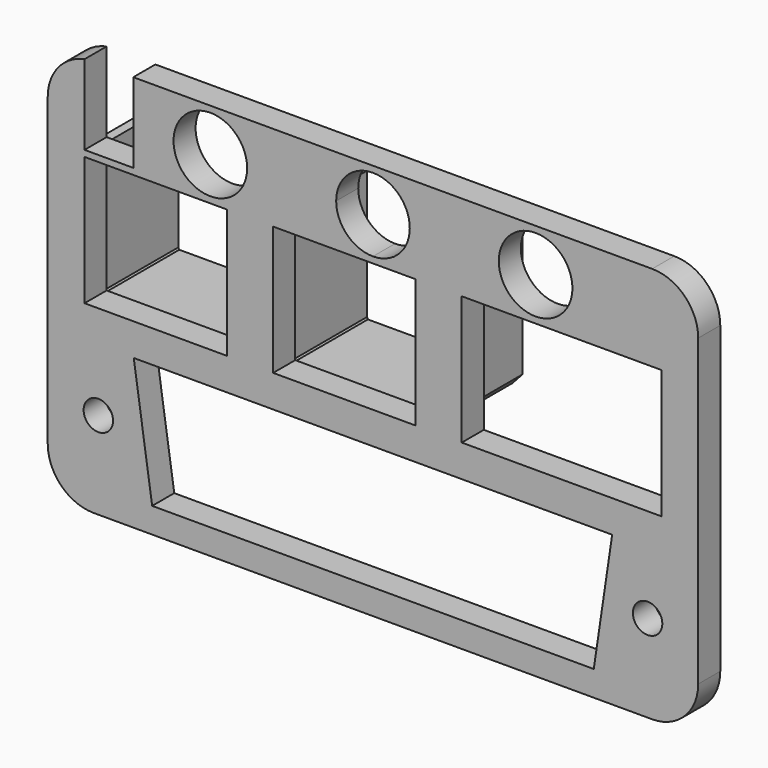
from build123d import *

# Parameters (mm, degrees)
F0_W        = 70.7
F0_H        = 43.1
F3_DEPTH    = 3
F1_R        = 1.6
F4_DEPTH    = 3
F2_W        = 15.5
F2_H        = 14
F2_W_2      = 5.3
F2_H_2      = 4
F2_H_3      = 4.6764186437
F2_W_3      = 21.7
F5_DEPTH    = 3
F6_T1_DEPTH = 27.4948974279
F6_T3_DEPTH = 28
F7_W        = 1
F7_H        = 14
F7_H_2      = 7
F7_W_2      = 15.7
F7_H_3      = 1
F8_DEPTH    = 10


# Not quite as in the source:
# - a fillet or chamfer that OpenCascade refuses, or shapes differently, is made with other operations: its cross-section is extruded or revolved along the edge and cut away or added


with BuildPart() as f3:
    # F0 (on Front) → F3 (new body)
    with BuildSketch(Plane.XZ):
        Rectangle(F0_W, F0_H)
    extrude(amount=F3_DEPTH)

    # F1 (on face) → F4 (cut)
    with BuildSketch(Plane.XZ):
        Polygon((0, -12.0528372875), (0, -18.8028372875), (24, -18.8028372875), (26, -5.3028372875), (0, -5.3028372875), align=None)
        Polygon((-24, -18.8028372875), (0, -18.8028372875), (0, -12.0528372875), (-25, -12.0528372875), align=None)
        with Locations((-29.85, -12.0528372875)):
            Circle(F1_R)
        Polygon((-25, -12.0528372875), (0, -12.0528372875), (0, -5.3028372875), (-26, -5.3028372875), align=None)
        with Locations((29.85, -12.0528372875)):
            Circle(F1_R)
    extrude(amount=F4_DEPTH, mode=Mode.SUBTRACT)

    # F2 (on face) → F5 (cut)
    with BuildSketch(Plane.XZ):
        with Locations((-23.6, 5.1971627125)):
            Rectangle(F2_W, F2_H)
        with Locations((-28.7, 14.8735813563)):
            Rectangle(F2_W_2, F2_H_2)
        with Locations((-28.7, 19.2117906781)):
            Rectangle(F2_W_2, F2_H_3)
        with BuildLine():
            ThreePointArc((-21.675, 16.8735813563), (-17.675, 12.8735813563), (-13.675, 16.8735813563))
            Line((-13.675, 16.8735813563), (-21.675, 16.8735813563))
        make_face()
        with BuildLine():
            Line((-21.675, 16.8735813563), (-13.675, 16.8735813563))
            ThreePointArc((-13.675, 16.8735813563), (-17.675, 20.8735813563), (-21.675, 16.8735813563))
        make_face()
        with BuildLine():
            ThreePointArc((21.675, 16.8735813563), (17.675, 20.8735813563), (13.675, 16.8735813563))
            Line((13.675, 16.8735813563), (21.675, 16.8735813563))
        make_face()
        with BuildLine():
            Line((21.675, 16.8735813563), (13.675, 16.8735813563))
            ThreePointArc((13.675, 16.8735813563), (17.675, 12.8735813563), (21.675, 16.8735813563))
        make_face()
        with BuildLine():
            ThreePointArc((-4, 16.8735813563), (-2.8284271247, 14.0451542315), (0, 12.8735813563))
            Line((0, 12.8735813563), (0, 16.8735813563))
            Line((0, 16.8735813563), (-4, 16.8735813563))
        make_face()
        with BuildLine():
            Line((0, 16.8735813563), (0, 12.8735813563))
            ThreePointArc((0, 12.8735813563), (2.8284271247, 14.0451542315), (4, 16.8735813563))
            Line((4, 16.8735813563), (0, 16.8735813563))
        make_face()
        with Locations((20.5, 5.1971627125)):
            Rectangle(F2_W_3, F2_H)
        Polygon((-10.85, 12.1971627125), (-10.85, -1.8028372875), (4.65, -1.8028372875), (4.65, 12.1971627125), (0, 12.1971627125), align=None)
        with BuildLine():
            Line((-4, 16.8735813563), (0, 16.8735813563))
            Line((0, 16.8735813563), (0, 20.8735813563))
            ThreePointArc((0, 20.8735813563), (-2.8284271247, 19.702008481), (-4, 16.8735813563))
        make_face()
        with BuildLine():
            Line((0, 20.8735813563), (0, 16.8735813563))
            Line((0, 16.8735813563), (4, 16.8735813563))
            ThreePointArc((4, 16.8735813563), (2.8284271247, 19.702008481), (0, 20.8735813563))
        make_face()
    extrude(amount=F5_DEPTH, mode=Mode.SUBTRACT)

    # F6: fillet of radius 5 on 4 edges, made by hand

    # F6_s2 → F6_t1 (cut)
    with BuildSketch(Plane.XZ.offset(-12.2474487139)):
        with BuildLine():
            ThreePointArc((-35.35, 16.6510205144), (-34.2229833462, 19.8132981746), (-31.35, 21.55))
            Line((-31.35, 21.55), (-35.35, 21.55))
            Line((-35.35, 21.55), (-35.35, 16.6510205144))
        make_face()
    extrude(amount=F6_T1_DEPTH, mode=Mode.SUBTRACT)

    # F6_s4 → F6_t3 (cut)
    with BuildSketch(Plane.XZ.offset(-12.5)):
        with BuildLine():
            ThreePointArc((35.35, 16.55), (33.8855339059, 20.0855339059), (30.35, 21.55))
            Line((30.35, 21.55), (35.35, 21.55))
            Line((35.35, 21.55), (35.35, 16.55))
        make_face()
        with BuildLine():
            ThreePointArc((30.35, -21.55), (33.8855339059, -20.0855339059), (35.35, -16.55))
            Line((35.35, -16.55), (35.35, -21.55))
            Line((35.35, -21.55), (30.35, -21.55))
        make_face()
        with BuildLine():
            ThreePointArc((-35.35, -16.55), (-33.8855339059, -20.0855339059), (-30.35, -21.55))
            Line((-30.35, -21.55), (-35.35, -21.55))
            Line((-35.35, -21.55), (-35.35, -16.55))
        make_face()
    extrude(amount=F6_T3_DEPTH, mode=Mode.SUBTRACT)

    # F7 (on face) → F8 (join)
    with BuildSketch(Plane(origin=(0, 0, 0), x_dir=(-1, 0, 0), z_dir=(0, 1, 0))):
        Polygon((15.75, -2.0028372875), (15.75, -3.0028372875), (31.45, -3.0028372875), (31.45, -2.0028372875), (23.6, -2.0028372875), align=None)
        Polygon((31.45, -2.0028372875), (31.45, -3.0028372875), (32.55, -1.8028372875), (31.55, -1.8028372875), align=None)
        with Locations((32.05, 5.1971627125)):
            Rectangle(F7_W, F7_H)
        Polygon((14.65, -1.8028372875), (15.75, -3.0028372875), (15.75, -2.0028372875), (15.65, -1.8028372875), align=None)
        with Locations((15.15, 1.6971627125)):
            Rectangle(F7_W, F7_H_2)
        with Locations((15.15, 8.6971627125)):
            Rectangle(F7_W, F7_H_2)
        with Locations((3.1, -2.5028372875)):
            Rectangle(F7_W_2, F7_H_3)
        Polygon((-5.85, -1.8028372875), (-4.75, -3.0028372875), (-4.75, -2.0028372875), (-4.85, -1.8028372875), align=None)
        with Locations((-5.35, 5.1971627125)):
            Rectangle(F7_W, F7_H)
        with Locations((11.55, 1.6971627125)):
            Rectangle(F7_W, F7_H_2)
        with Locations((11.55, 8.6971627125)):
            Rectangle(F7_W, F7_H_2)
        Polygon((10.95, -3.0028372875), (12.05, -1.8028372875), (11.05, -1.8028372875), (10.95, -2.0028372875), align=None)
    extrude(amount=F8_DEPTH)


solid = f3.part
